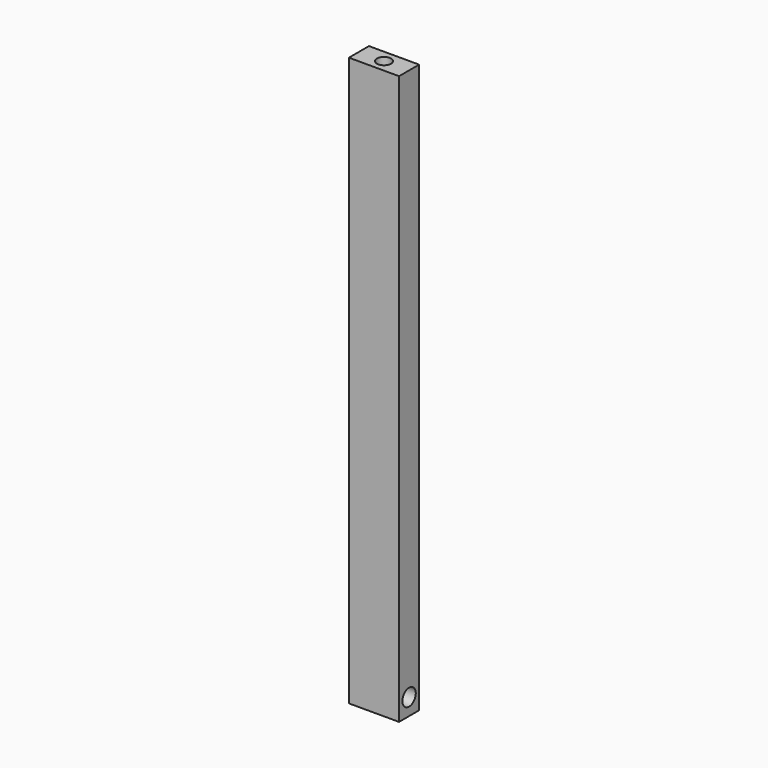
from build123d import *

# Parameters (mm, degrees)
F0_W     = 38.1
F0_H     = 431.8
F1_DEPTH = 9.525
F3_D     = 12.7
F5_D     = 10.71626
F5_DEPTH = 38.0941384615
F5_TIP   = 3.2194893086


# Not quite as in the source:
# - a length typed as a fraction of an inch, garbled in the dataset ("3 / 203.2 mm" for 3/8 in), is restored


with BuildPart() as f1:
    # F0 (on Front) → F1 (new body, symmetric)
    with BuildSketch(Plane.XZ):
        Rectangle(F0_W, F0_H)
    extrude(amount=F1_DEPTH, both=True)

    # F3 (through all)
    with Locations(Plane.YZ.offset(19.05)):
        with Locations((0, -203.2)):
            Hole(F3_D / 2)

    # F5
    with Locations(Plane.XY.offset(215.9)):
        with Locations((0, 0)):
            Hole(F5_D / 2, depth=F5_DEPTH)
            with Locations((0, 0, -(F5_DEPTH + F5_TIP / 2))):  # 118° drill point
                Cone(0, F5_D / 2, F5_TIP, mode=Mode.SUBTRACT)


solid = f1.part
